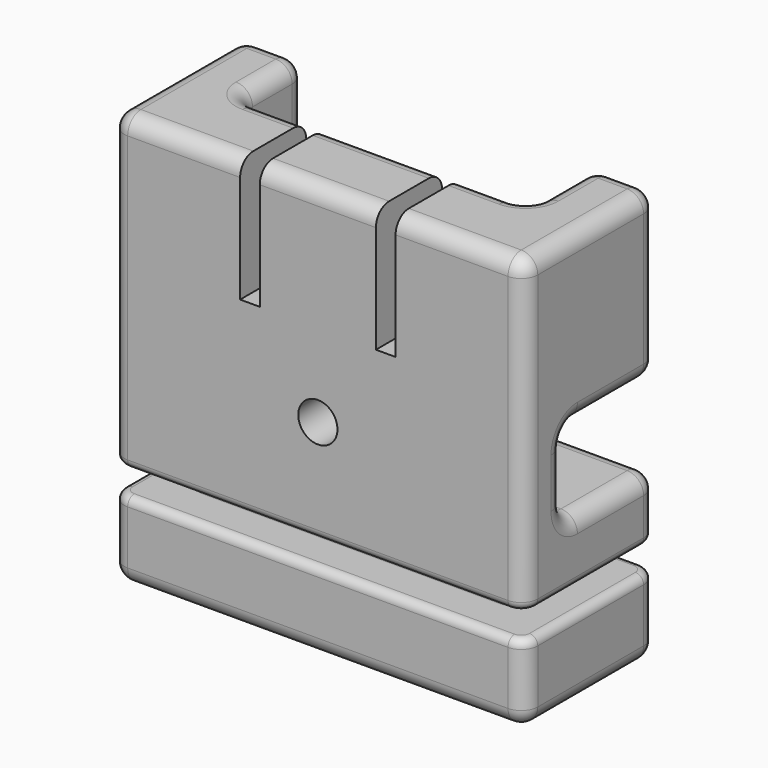
from build123d import *

# Parameters (mm, degrees)
F0_W      = 50
F0_H      = 50
F1_DEPTH  = 10
F2_W      = 14
F2_H      = 10
F3_DEPTH  = 76.70555
F4_F1_R   = 2
F4_F2_R   = 2
F5_W      = 13.7121686712
F5_H      = 20
F6_DEPTH  = 17.5
F7_R      = 2
F8_W      = 3
F8_H      = 5.7575751543
F9_DEPTH  = 29.7216
F10_R     = 1
F11_W     = 46
F11_H     = 3
F11_W_2   = 2
F12_DEPTH = 6
F13_W     = 7.5689357519
F13_H     = 3
F13_W_2   = 12
F14_DEPTH = 6
F15_W     = 8.5923536867
F15_H     = 3
F15_W_2   = 42
F16_DEPTH = 6
F17_W     = 8
F17_H     = 3
F18_DEPTH = 6
F19_R     = 1
F20_R     = 2.3714715185
F21_DEPTH = 25
F23_W     = 2.3758355528
F23_H     = 10
F24_DEPTH = 40


with BuildPart() as f1:
    # F0 (on Front) → F1 (new body, symmetric)
    with BuildSketch(Plane.XZ):
        Rectangle(F0_W, F0_H)
    extrude(amount=F1_DEPTH, both=True)

    # F2 (on face) → F3 (cut)
    with BuildSketch(Plane.YZ.offset(25)):
        with Locations((3, 0)):
            Rectangle(F2_W, F2_H)
    extrude(amount=-F3_DEPTH, mode=Mode.SUBTRACT)

    # F4: fillet of radius 2 on 20 edges, made by hand

    # F4_f1
    f4_f1_edges = [f1.edges().sort_by_distance(p)[0] for p in [
        (0, -4, -5),
        (0, -4, 5),
    ]]
    fillet(f4_f1_edges, radius=F4_F1_R)

    # F4_f2
    f4_f2_edges = [f1.edges().sort_by_distance(p)[0] for p in [
        (0, 10, 25),
        (0, -10, 25),
        (0, 10, -5),
        (0, 10, -25),
        (0, -10, -25),
        (25, -10, 0),
        (25, 10, -15),
        (-25, 10, -15),
        (-25, -10, 0),
        (-25, 10, 15),
        (-25, 0, 25),
        (25, 0, 25),
        (25, 10, 15),
        (25, 4, -5),
        (0, 10, 5),
        (-25, 4, 5),
        (-25, 0, -25),
        (25, 0, -25),
        (-25, -3.4142135624, 4.4142135624),
        (25, -3.4142135624, -4.4142135624),
    ]]
    fillet(f4_f2_edges, radius=F4_F2_R)

    # F5 (on Right) → F6 (cut, symmetric)
    with BuildSketch(Plane.YZ):
        with Locations((6.8560843356, 20)):
            Rectangle(F5_W, F5_H)
    extrude(amount=F6_DEPTH, both=True, mode=Mode.SUBTRACT)

    # F7
    f7_edges = [f1.edges().sort_by_distance(p)[0] for p in [
        (0, 0, 10),
        (0, 0, 25),
        (17.5, 4, 25),
        (17.5, 5, 10),
        (0, 10, 10),
        (-17.5, 5, 10),
        (-17.5, 0, 17.5),
        (17.5, 0, 17.5),
        (-17.5, 10, 16.5),
        (17.5, 10, 16.5),
        (-17.5, 9.414214, 24.414214),
        (17.5, 9.414214, 24.414214),
    ]]
    fillet(f7_edges, radius=F7_R)

    # F8 (on Top) → F9 (cut)
    with BuildSketch(Plane.XY):
        with Locations((3.5149400131, 8.914668113)):
            Rectangle(F8_W, F8_H)
        with Locations((-3.5149400131, 8.914668113)):
            Rectangle(F8_W, F8_H)
    extrude(amount=F9_DEPTH, mode=Mode.SUBTRACT)

    # F10
    f10_edges = [f1.edges().sort_by_distance(p)[0] for p in [
        (3.51494, 6.035881, 10),
        (2.01494, 6.035881, 7.5),
        (2.01494, 7.01794, 10),
        (-3.51494, 6.035881, 10),
        (-5.01494, 7.01794, 10),
        (3.51494, 6.035881, 5),
        (5.01494, 6.035881, 7.5),
        (5.01494, 9.414214, 5.585786),
        (-2.01494, 7.01794, 5),
        (-3.51494, 6.035881, 5),
        (-2.01494, 6.035881, 7.5),
        (-5.01494, 6.035881, 7.5),
    ]]
    fillet(f10_edges, radius=F10_R)

    # F11 (on face) → F12 (cut)
    with BuildSketch(Plane(origin=(0, 10, 0), x_dir=(-1, 0, 0), z_dir=(0, 1, 0))):
        with Locations((0, -14)):
            Rectangle(F11_W, F11_H)
        with Locations((-24, -14)):
            Rectangle(F11_W_2, F11_H)
        with Locations((24, -14)):
            Rectangle(F11_W_2, F11_H)
    extrude(amount=-F12_DEPTH, mode=Mode.SUBTRACT)

    # F13 (on face) → F14 (cut)
    with BuildSketch(Plane.YZ.offset(25)):
        with Locations((-11.784467876, -14)):
            Rectangle(F13_W, F13_H)
        with Locations((-2, -14)):
            Rectangle(F13_W_2, F13_H)
    extrude(amount=-F14_DEPTH, mode=Mode.SUBTRACT)

    # F15 (on face) → F16 (cut)
    with BuildSketch(Plane.XZ.offset(10)):
        with Locations((-27.2961768433, -14)):
            Rectangle(F15_W, F15_H)
        with Locations((-2, -14)):
            Rectangle(F15_W_2, F15_H)
    extrude(amount=-F16_DEPTH, mode=Mode.SUBTRACT)

    # F17 (on face) → F18 (cut)
    with BuildSketch(Plane(origin=(-25, 0, 0), x_dir=(0, -1, 0), z_dir=(-1, 0, 0))):
        with Locations((0, -14)):
            Rectangle(F17_W, F17_H)
        Polygon((8, -12.5), (4, -12.5), (4, -15.5), (8, -15.5), (13.1623027846, -15.5), (13.1623027846, -12.5), align=None)
    extrude(amount=-F18_DEPTH, mode=Mode.SUBTRACT)

    # F19
    f19_edges = [f1.edges().sort_by_distance(p)[0] for p in [
        (0, 10, -15.5),
        (0, 4, -15.5),
        (19, 0, -12.5),
        (0, 4, -12.5),
        (0, 10, -12.5),
        (24.414214, 9.414214, -12.5),
        (25, 0, -12.5),
        (19, 4, -14),
        (19, 0, -15.5),
        (25, 0, -15.5),
        (24.414214, 9.414214, -15.5),
        (24.414214, -9.414214, -15.5),
        (0, -4, -15.5),
        (0, -10, -15.5),
        (0, -4, -12.5),
        (0, -10, -12.5),
        (-19, 0, -12.5),
        (-25, 0, -12.5),
        (-24.414214, -9.414214, -12.5),
        (-19, -4, -14),
        (-19, 4, -14),
        (-19, 0, -15.5),
        (-24.414214, 9.414214, -15.5),
        (-25, 0, -15.5),
        (-24.414214, -9.414214, -15.5),
        (-24.414214, 9.414214, -12.5),
        (19, -4, -14),
        (24.414214, -9.414214, -12.5),
    ]]
    fillet(f19_edges, radius=F19_R)

    # F20 (on face) → F21 (cut)
    with BuildSketch(Plane(origin=(0, -4, 0), x_dir=(-1, 0, 0), z_dir=(0, 1, 0))):
        Circle(F20_R)
    extrude(amount=-F21_DEPTH, mode=Mode.SUBTRACT)

    # F23 (on offset) → F24 (cut)
    with BuildSketch(Plane.XY.offset(50)):
        with Locations((8.2101970911, -5)):
            Rectangle(F23_W, F23_H)
        with Locations((-8.2101970911, -5)):
            Rectangle(F23_W, F23_H)
    extrude(amount=-F24_DEPTH, mode=Mode.SUBTRACT)


solid = f1.part
